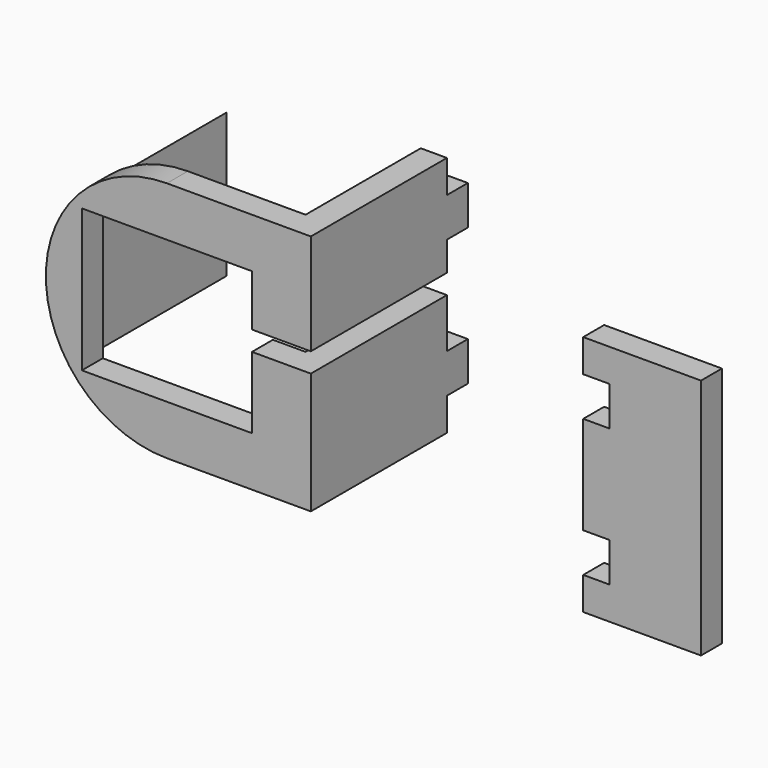
from build123d import *

# Parameters (mm, degrees)
F0_W     = 2
F0_H     = 2.5
F0_H_2   = 3
F0_H_3   = 2.2283997163
F0_H_4   = 3.7716002837
F1_DEPTH = 2
F0_H_5   = 7.5
F2_DEPTH = 13
F3_DEPTH = 11


# Not quite as in the source:
# - a feature names something its author has since deleted; it is built from what else it names


with BuildPart() as f1:
    # F0 (on Front) → F1 (new body)
    with BuildSketch(Plane.XZ):
        Polygon((27.9331561178, 18.5), (27.9331561178, 14.7), (34.4331561178, 14.7), (34.4331561178, 10.7716002837), (36.9331561178, 10.7716002837), (36.9331561178, 13), (36.9331561178, 16), (36.9331561178, 18.5), align=None)
        with BuildLine():
            ThreePointArc((20.4959187275, 3.75), (23.7685733056, 0.9905357317), (27.9331561178, 0))
            Line((27.9331561178, 0), (27.9331561178, 3.8))
            Line((27.9331561178, 3.8), (21.4331561178, 3.8))
            Line((21.4331561178, 3.8), (21.4331561178, 14.7))
            Line((21.4331561178, 14.7), (27.9331561178, 14.7))
            Line((27.9331561178, 14.7), (27.9331561178, 18.5))
            ThreePointArc((27.9331561178, 18.5), (23.7685733056, 17.5094642683), (20.4959187275, 14.75))
            Line((20.4959187275, 14.75), (20.4959187275, 3.75))
        make_face()
        Polygon((27.9331561178, 3.8), (27.9331561178, 0), (36.9331561178, 0), (36.9331561178, 2.5), (36.9331561178, 5.5), (36.9331561178, 9.2716002837), (34.4331561178, 9.2716002837), (34.4331561178, 3.8), align=None)
        with Locations((37.9331561178, 17.25)):
            Rectangle(F0_W, F0_H)
        with Locations((37.9331561178, 14.5)):
            Rectangle(F0_W, F0_H_2)
        with Locations((37.9331561178, 11.8858001418)):
            Rectangle(F0_W, F0_H_3)
        with Locations((37.9331561178, 7.3858001418)):
            Rectangle(F0_W, F0_H_4)
        with Locations((37.9331561178, 4)):
            Rectangle(F0_W, F0_H_2)
        with Locations((37.9331561178, 1.25)):
            Rectangle(F0_W, F0_H)
        with BuildLine():
            ThreePointArc((20.4959187275, 14.75), (18.6831561178, 9.25), (20.4959187275, 3.75))
            Line((20.4959187275, 3.75), (20.4959187275, 14.75))
        make_face()
    extrude(amount=F1_DEPTH)

    # F0 (on Front) → F2 (join)
    with BuildSketch(Plane.XZ):
        with Locations((37.9331561178, 14.5)):
            Rectangle(F0_W, F0_H_2)
        with Locations((37.9331561178, 4)):
            Rectangle(F0_W, F0_H_2)
        with BuildLine():
            ThreePointArc((20.4959187275, 14.75), (18.6831561178, 9.25), (20.4959187275, 3.75))
            Line((20.4959187275, 3.75), (20.4959187275, 14.75))
        make_face()
    extrude(amount=-F2_DEPTH)

    # F0 (on Front) → F3 (join)
    with BuildSketch(Plane.XZ):
        with Locations((37.9331561178, 17.25)):
            Rectangle(F0_W, F0_H)
        with Locations((37.9331561178, 11.8858001418)):
            Rectangle(F0_W, F0_H_3)
        with Locations((37.9331561178, 7.3858001418)):
            Rectangle(F0_W, F0_H_4)
        with Locations((37.9331561178, 1.25)):
            Rectangle(F0_W, F0_H)
    extrude(amount=-F3_DEPTH)


with BuildPart() as f1b:
    # F0 (on Front) → F1, piece 2 (new body)
    with BuildSketch(Plane.XZ):
        Polygon((68.7529053539, 18.5), (61.7529053539, 18.5), (61.7529053539, 16), (61.7529053539, 13), (61.7529053539, 5.5), (61.7529053539, 2.5), (61.7529053539, 0), (68.7529053539, 0), align=None)
        with Locations((60.7529053539, 17.25)):
            Rectangle(F0_W, F0_H)
        with Locations((60.7529053539, 9.25)):
            Rectangle(F0_W, F0_H_5)
        with Locations((60.7529053539, 1.25)):
            Rectangle(F0_W, F0_H)
    extrude(amount=F1_DEPTH)


solid = Compound([f1.part, f1b.part])
